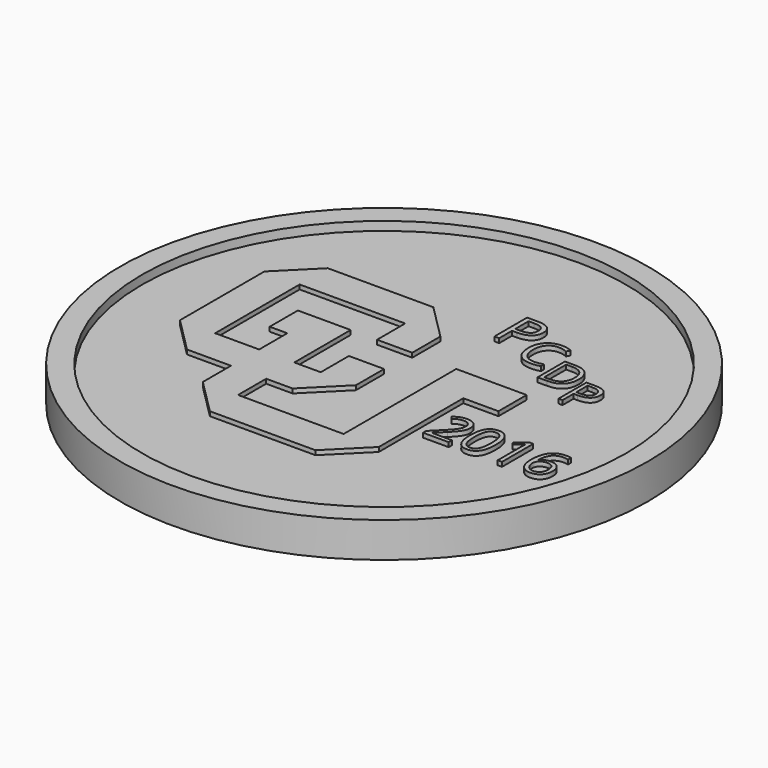
from build123d import *

# Parameters (mm, degrees)
F0_R           = 38.1
F1_DEPTH       = 3.81
F2_R           = 38.1
F2_R_2         = 34.925
F3_DEPTH       = 0.635
F5_TEXT_SIZE   = 8.2517766497
F5_TEXT_SIZE_2 = 7.6283435007
F5_TEXT_SIZE_3 = 6.932196162
F5_TEXT_SIZE_4 = 7.0555555556
F3_FACE_R      = 38.1
F3_FACE_R_2    = 34.925
F6_DEPTH       = 0.635
F8_TEXT_SIZE   = 14.2819211246
F8_TEXT_SIZE_2 = 14.1111111111
F9_DEPTH       = 0.635
F10_TEXT_SIZE  = 7.8950785044
F11_DEPTH      = 0.635


# Not quite as in the source:
# - the program builds the solid bodies; features that only make, move or delete a surface that nothing else refers to are left out
# - Text() gives the source's letters only with a copy of the font that has no kerning and outlines rounded to 1/6400 em; it was checked with that copy


with BuildPart() as f1:
    # F0 (on Top) → F1 (new body)
    with BuildSketch(Plane.XY):
        Circle(F0_R)
    extrude(amount=F1_DEPTH)

    # F2 (on face) → F3 (join)
    with BuildSketch(Plane.XY.offset(3.81)):
        Circle(F2_R)
        Circle(F2_R_2, mode=Mode.SUBTRACT)
        Polygon((0, -5.08), (0, 0), (-5.08, 0), (-5.08, -5.08), (-8.89, -5.08), (-8.89, 5.08), (-16.51, 5.08), (-16.51, 0), (-13.97, 0), (-13.97, -5.08), (-20.32, -5.08), (-20.32, 10.16), (-5.08, 10.16), (-5.08, 5.08), (0, 5.08), (0, 10.16), (-5.08, 15.24), (-20.32, 15.24), (-25.4, 10.16), (-25.4, -5.08), (-20.32, -10.16), (-13.97, -10.16), (-13.97, -15.24), (-8.89, -20.32), (6.35, -20.32), (11.43, -15.24), (11.43, 0), (16.51, 0), (16.51, 5.08), (6.35, 5.08), (6.35, -15.24), (-8.89, -15.24), (-8.89, -10.16), (-5.08, -10.16), align=None)
    extrude(amount=F3_DEPTH)

    # F5 (on face) + F3_face (on face) → F6 (join)
    with BuildSketch(Plane.XY.offset(3.81)):
        with Locations((3.9412065944, 13.9769603866)):
            Text('P', F5_TEXT_SIZE, font='Open Sans', text_align=(TextAlign.LEFT, TextAlign.BOTTOM))
        with Locations((9.0212065944, 11.45519266)):
            Text('C', F5_TEXT_SIZE_2, font='Open Sans', text_align=(TextAlign.LEFT, TextAlign.BOTTOM))
        with Locations((14.1012065944, 9.2102150835)):
            Text('D', F5_TEXT_SIZE_3, font='Open Sans', text_align=(TextAlign.LEFT, TextAlign.BOTTOM))
        with Locations((19.1812065944, 6.6258057019)):
            Text('P', F5_TEXT_SIZE_4, font='Open Sans', text_align=(TextAlign.LEFT, TextAlign.BOTTOM))
    with BuildSketch(Plane.XY.offset(4.445)):
        Circle(F3_FACE_R)
        Circle(F3_FACE_R_2, mode=Mode.SUBTRACT)
    extrude(amount=F6_DEPTH)

    # F8 (on face) → F9 (join)
    with BuildSketch(Plane(origin=(0, 0, 0), x_dir=(1, 0, 0), z_dir=(0, 0, -1))):
        with Locations((-28.676790696, 4.8278645518)):
            Text('Robert', F8_TEXT_SIZE, font='Open Sans', text_align=(TextAlign.LEFT, TextAlign.BOTTOM))
        with Locations((-15.1301199583, -5.3321354482)):
            Text('Jones', F8_TEXT_SIZE_2, font='Open Sans', text_align=(TextAlign.LEFT, TextAlign.BOTTOM))
    extrude(amount=F9_DEPTH)

    # F10 (on face) → F11 (join)
    with BuildSketch(Plane.XY.offset(3.81)):
        with Locations((12.7602651688, -9.40431673)):
            Text('2016', F10_TEXT_SIZE, font='Open Sans', text_align=(TextAlign.LEFT, TextAlign.BOTTOM))
    extrude(amount=F11_DEPTH)


solid = f1.part
